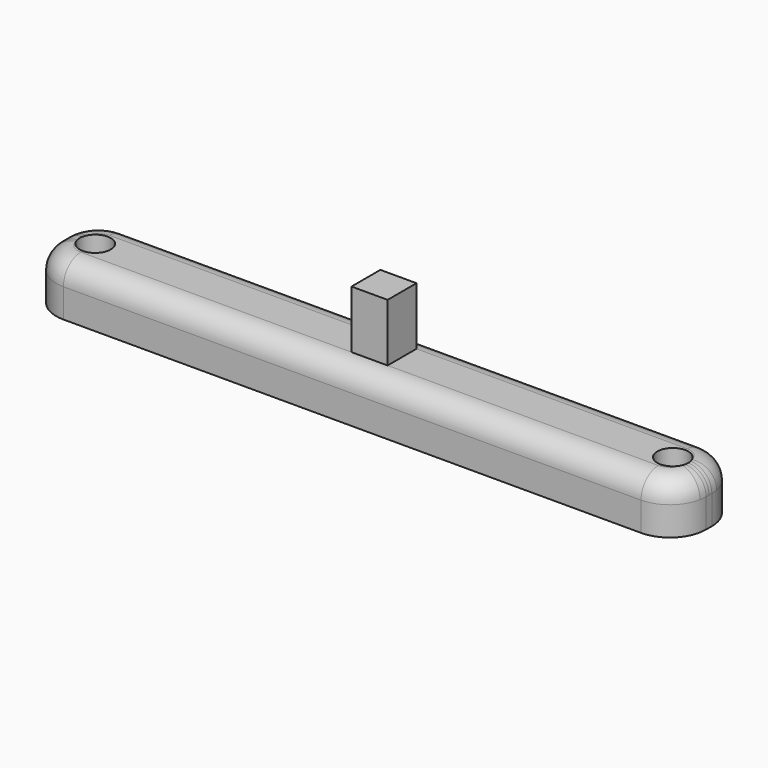
from build123d import *

# Parameters (mm, degrees)
F0_W     = 90
F0_H     = 11
F0_R     = 2.15
F0_R_2   = 2.25
F1_DEPTH = 7
F2_W     = 5
F2_H     = 5
F3_DEPTH = 8
F4_R     = 5
F5_R     = 2.99999


# Not quite as in the source:
# - a fillet or chamfer is up to 0.001 mm smaller than in the source, because OpenCascade refuses the exact size


with BuildPart() as f1:
    # F0 (on Top) → F1 (new body)
    with BuildSketch(Plane.XY):
        Rectangle(F0_W, F0_H)
        with Locations((-40, 0)):
            Circle(F0_R, mode=Mode.SUBTRACT)
        Circle(F0_R_2, mode=Mode.SUBTRACT)
        with Locations((40, 0)):
            Circle(F0_R, mode=Mode.SUBTRACT)
        Circle(F0_R_2)
    extrude(amount=F1_DEPTH)

    # F2 (on face) → F3 (join)
    with BuildSketch(Plane.XY.offset(7)):
        Rectangle(F2_W, F2_H)
    extrude(amount=F3_DEPTH)

    # F4
    f4_edges = [f1.edges().sort_by_distance(p)[0] for p in [
        (45, -5.5, 3.5),
        (45, 5.5, 3.5),
        (-45, -5.5, 3.5),
        (-45, 5.5, 3.5),
    ]]
    fillet(f4_edges, radius=F4_R)

    # F5 (radius 3 in the source; OpenCascade refuses exactly that, so slightly less here)
    f5_edges = [f1.edges().sort_by_distance(p)[0] for p in [
        (0, -5.5, 7),
    ]]
    fillet(f5_edges, radius=F5_R)


solid = f1.part
